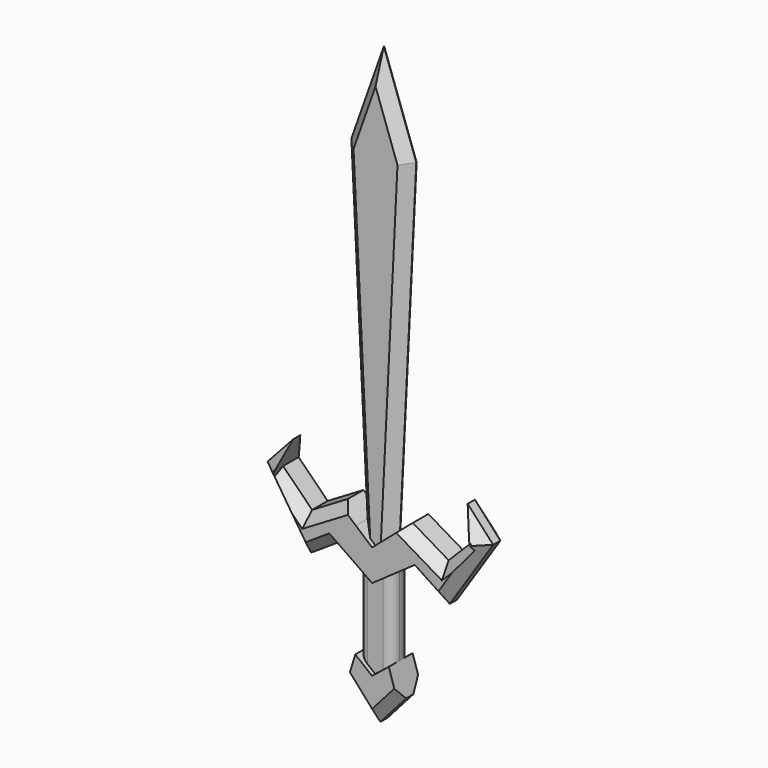
from build123d import *

# Parameters (mm, degrees)
F1_DEPTH      = 2.33167
F2_SIZE       = 2.286
F3_DEPTH      = 3.27792
F4_T4_DEPTH   = 23.2837004238
F4_T9_DEPTH   = 15.3016603011
F4_T14_DEPTH  = 15.3016603011
F4_T19_DEPTH  = 23.2837004238
F4_T24_DEPTH  = 23.2837004238
F4_T29_DEPTH  = 15.3016603011
F4_T34_DEPTH  = 23.2837004238
F4_T39_DEPTH  = 15.3016603011
F4_T44_DEPTH  = 20.0662153039
F4_T50_DEPTH  = 20.0662153039
F4_T56_DEPTH  = 20.0662153039
F4_T62_DEPTH  = 20.0662153039
F4_T68_DEPTH  = 20.8098338881
F4_T74_DEPTH  = 20.9196420642
F4_T80_DEPTH  = 20.9196420642
F4_T86_DEPTH  = 20.8098338881
F4_T93_DEPTH  = 20.0662153039
F4_T97_DEPTH  = 23.2837004238
F4_T104_DEPTH = 29.1625677342
F4_T108_DEPTH = 21.1805276116
F4_T115_DEPTH = 21.1805276116
F4_T119_DEPTH = 29.1625677342
F4_T126_DEPTH = 23.2837004238
F4_T130_DEPTH = 20.0662153039
F4_T137_DEPTH = 20.0662153039
F4_T141_DEPTH = 23.2837004238
F4_T148_DEPTH = 29.1625677342
F4_T152_DEPTH = 21.1805276116
F4_T159_DEPTH = 21.1805276116
F4_T163_DEPTH = 29.1625677342
F4_T170_DEPTH = 23.2837004238
F4_T174_DEPTH = 20.0662153039
F4_T181_DEPTH = 20.8098338881
F4_T185_DEPTH = 20.9196420642
F4_T192_DEPTH = 20.9196420642
F4_T196_DEPTH = 20.8098338881
F5_DEPTH      = 2.39562
F6_R          = 2.032
F7_DEPTH      = 3.2766
F8_SIZE       = 2.286


# Not quite as in the source:
# - a fillet or chamfer that OpenCascade refuses, or shapes differently, is made with other operations: its cross-section is extruded or revolved along the edge and cut away or added


with BuildPart() as f1:
    # F0 (on Front) → F1 (new body, symmetric)
    with BuildSketch(Plane.XZ):
        Polygon((0, -27.3264925927), (3.569676308, -24.2491848767), (7.1393526159, 48.2521876693), (0, 68.4393197298), (-7.1393526159, 48.2521876693), (-3.569676308, -24.2491848767), align=None)
    extrude(amount=F1_DEPTH, both=True)

    # F2
    f2_edges = [f1.edges().sort_by_distance(p)[0] for p in [
        (-5.354514, -2.33167, 12.001501),
        (5.354514, -2.33167, 12.001501),
        (-3.569676, -2.33167, 58.345754),
        (3.569676, -2.33167, 58.345754),
        (-3.569676, 2.33167, 58.345754),
        (3.569676, 2.33167, 58.345754),
        (5.354514, 2.33167, 12.001501),
        (-5.354514, 2.33167, 12.001501),
    ]]
    chamfer(f2_edges, length=F2_SIZE)

    # F0 (on Front) → F3 (join, symmetric)
    with BuildSketch(Plane.XZ):
        Polygon((-3.6927689798, -31.6347228363), (0, -34.2196598649), (3.6927689798, -31.6347228363), (7.3855379596, -29.0497858077), (15.2634456754, -34.2196598649), (24.812715756, -19.6683830609), (19.2023981363, -13.540154323), (21.41806297, -19.4485839456), (15.01726266, -25.849385187), (7.1393526159, -21.1718771607), (3.569676308, -24.2491848767), (0, -27.3264925927), (-3.569676308, -24.2491848767), (-7.1393526159, -21.1718771607), (-15.01726266, -25.849385187), (-21.41806297, -19.4485839456), (-19.2023981363, -13.540154323), (-24.812715756, -19.6683830609), (-15.2634456754, -34.2196598649), (-7.3855379596, -29.0497858077), align=None)
    extrude(amount=F3_DEPTH, both=True)

    # F4: chamfer of 2.286 on 16 edges, made by hand


with BuildPart() as f4_tool2:
    # F4_s3 → F4_t4 (new body)
    with BuildSketch(Plane(origin=(-1.6727458566, 0, 2.5489474878), x_dir=(0, 1, 0), z_dir=(0.5486562278, 0, -0.8360480511))):
        with BuildLine():
            Line((-3.3425778441, -29.1851456624), (-0.9272621559, -31.6004613506))
            Line((-0.9272621559, -31.6004613506), (-0.9272621559, -31.6461813506))
            ThreePointArc((-0.9272621559, -31.6461813506), (-2.102591078, -31.5815235065), (-3.27792, -31.5815235065))
            Line((-3.27792, -31.5815235065), (-3.32364, -31.5358035065))
            ThreePointArc((-3.32364, -31.5358035065), (-3.32364, -30.3604745845), (-3.3882978441, -29.1851456624))
            Line((-3.3882978441, -29.1851456624), (-3.3425778441, -29.1851456624))
        make_face()
    extrude(amount=F4_T4_DEPTH)

    split(bisect_by=Plane(origin=(-3.7030026198, 0, 3.3900531022), x_dir=(0, 1, 0), z_dir=(0.7375871681, 0, -0.6752519304)), keep=Keep.TOP)


with BuildPart() as f1_1:
    add(f1.part)

    # F4_t1: cut F4_tool2
    add(f4_tool2.part, mode=Mode.SUBTRACT)


with BuildPart() as f4_tool7:
    # F4_s8 → F4_t9 (new body)
    with BuildSketch(Plane(origin=(-26.3654470614, 0, -17.3023149911), x_dir=(0, 1, 0), z_dir=(0.8360480511, 0, 0.5486562278))):
        with BuildLine():
            Line((-3.3425778441, -17.8842375684), (-0.9272621559, -20.2995532566))
            Line((-0.9272621559, -20.2995532566), (-0.9272621559, -20.3452732566))
            ThreePointArc((-0.9272621559, -20.3452732566), (-2.102591078, -20.2806154125), (-3.27792, -20.2806154125))
            Line((-3.27792, -20.2806154125), (-3.32364, -20.2348954125))
            ThreePointArc((-3.32364, -20.2348954125), (-3.32364, -19.0595664905), (-3.3882978441, -17.8842375684))
            Line((-3.3882978441, -17.8842375684), (-3.3425778441, -17.8842375684))
        make_face()
    extrude(amount=F4_T9_DEPTH)

    split(bisect_by=Plane(origin=(-16.0763475957, 0, -22.9662220215), x_dir=(0, 1, 0), z_dir=(-0.5734621572, 0, -0.8192320516)), keep=Keep.TOP)


with BuildPart() as f1_2:
    add(f1_1.part)

    # F4_t6: cut F4_tool7
    add(f4_tool7.part, mode=Mode.SUBTRACT)


with BuildPart() as f4_tool12:
    # F4_s13 → F4_t14 (new body)
    with BuildSketch(Plane(origin=(13.5725237881, 0, -8.9069637719), x_dir=(0, 1, 0), z_dir=(0.8360480511, 0, -0.5486562278))):
        with BuildLine():
            Line((-3.3425778441, -17.8842375684), (-0.9272621559, -20.2995532566))
            Line((-0.9272621559, -20.2995532566), (-0.9272621559, -20.3452732566))
            ThreePointArc((-0.9272621559, -20.3452732566), (-2.102591078, -20.2806154125), (-3.27792, -20.2806154125))
            Line((-3.27792, -20.2806154125), (-3.32364, -20.2348954125))
            ThreePointArc((-3.32364, -20.2348954125), (-3.32364, -19.0595664905), (-3.3882978441, -17.8842375684))
            Line((-3.3882978441, -17.8842375684), (-3.3425778441, -17.8842375684))
        make_face()
    extrude(amount=F4_T14_DEPTH)

    split(bisect_by=Plane(origin=(16.0763475957, 0, -22.9662220215), x_dir=(0, 1, 0), z_dir=(0.5734621572, 0, -0.8192320516)), keep=Keep.TOP)


with BuildPart() as f1_3:
    add(f1_2.part)

    # F4_t11: cut F4_tool12
    add(f4_tool12.part, mode=Mode.SUBTRACT)


with BuildPart() as f4_tool17:
    # F4_s18 → F4_t19 (new body)
    with BuildSketch(Plane(origin=(-11.102001386, 0, -16.9173448738), x_dir=(0, 1, 0), z_dir=(0.5486562278, 0, 0.8360480511))):
        with BuildLine():
            Line((-3.3425778441, -29.1851456624), (-0.9272621559, -31.6004613506))
            Line((-0.9272621559, -31.6004613506), (-0.9272621559, -31.6461813506))
            ThreePointArc((-0.9272621559, -31.6461813506), (-2.102591078, -31.5815235065), (-3.27792, -31.5815235065))
            Line((-3.27792, -31.5815235065), (-3.32364, -31.5358035065))
            ThreePointArc((-3.32364, -31.5358035065), (-3.32364, -30.3604745845), (-3.3882978441, -29.1851456624))
            Line((-3.3882978441, -29.1851456624), (-3.3425778441, -29.1851456624))
        make_face()
    extrude(amount=F4_T19_DEPTH)

    split(bisect_by=Plane(origin=(3.7030026198, 0, 3.3900531022), x_dir=(0, 1, 0), z_dir=(-0.7375871681, 0, -0.6752519304)), keep=Keep.TOP)


with BuildPart() as f1_4:
    add(f1_3.part)

    # F4_t16: cut F4_tool17
    add(f4_tool17.part, mode=Mode.SUBTRACT)


with BuildPart() as f4_tool22:
    # F4_s23 → F4_t24 (new body)
    with BuildSketch(Plane(origin=(-1.6727458566, 0, 2.5489474878), x_dir=(0, 1, 0), z_dir=(0.5486562278, 0, -0.8360480511))):
        with BuildLine():
            Line((3.3425778441, -29.1851456624), (0.9272621559, -31.6004613506))
            Line((0.9272621559, -31.6004613506), (0.9272621559, -31.6461813506))
            ThreePointArc((0.9272621559, -31.6461813506), (2.102591078, -31.5815235065), (3.27792, -31.5815235065))
            Line((3.27792, -31.5815235065), (3.32364, -31.5358035065))
            ThreePointArc((3.32364, -31.5358035065), (3.32364, -30.3604745845), (3.3882978441, -29.1851456624))
            Line((3.3882978441, -29.1851456624), (3.3425778441, -29.1851456624))
        make_face()
    extrude(amount=F4_T24_DEPTH)

    split(bisect_by=Plane(origin=(-3.7030026198, 0, 3.3900531022), x_dir=(0, 1, 0), z_dir=(0.7375871681, 0, -0.6752519304)), keep=Keep.TOP)


with BuildPart() as f1_5:
    add(f1_4.part)

    # F4_t21: cut F4_tool22
    add(f4_tool22.part, mode=Mode.SUBTRACT)


with BuildPart() as f4_tool27:
    # F4_s28 → F4_t29 (new body)
    with BuildSketch(Plane(origin=(-26.3654470614, 0, -17.3023149911), x_dir=(0, 1, 0), z_dir=(0.8360480511, 0, 0.5486562278))):
        with BuildLine():
            Line((3.3425778441, -17.8842375684), (0.9272621559, -20.2995532566))
            Line((0.9272621559, -20.2995532566), (0.9272621559, -20.3452732566))
            ThreePointArc((0.9272621559, -20.3452732566), (2.102591078, -20.2806154125), (3.27792, -20.2806154125))
            Line((3.27792, -20.2806154125), (3.32364, -20.2348954125))
            ThreePointArc((3.32364, -20.2348954125), (3.32364, -19.0595664905), (3.3882978441, -17.8842375684))
            Line((3.3882978441, -17.8842375684), (3.3425778441, -17.8842375684))
        make_face()
    extrude(amount=F4_T29_DEPTH)

    split(bisect_by=Plane(origin=(-16.0763475957, 0, -22.9662220215), x_dir=(0, 1, 0), z_dir=(-0.5734621572, 0, -0.8192320516)), keep=Keep.TOP)


with BuildPart() as f1_6:
    add(f1_5.part)

    # F4_t26: cut F4_tool27
    add(f4_tool27.part, mode=Mode.SUBTRACT)


with BuildPart() as f4_tool32:
    # F4_s33 → F4_t34 (new body)
    with BuildSketch(Plane(origin=(-11.102001386, 0, -16.9173448738), x_dir=(0, 1, 0), z_dir=(0.5486562278, 0, 0.8360480511))):
        with BuildLine():
            Line((3.3425778441, -29.1851456624), (0.9272621559, -31.6004613506))
            Line((0.9272621559, -31.6004613506), (0.9272621559, -31.6461813506))
            ThreePointArc((0.9272621559, -31.6461813506), (2.102591078, -31.5815235065), (3.27792, -31.5815235065))
            Line((3.27792, -31.5815235065), (3.32364, -31.5358035065))
            ThreePointArc((3.32364, -31.5358035065), (3.32364, -30.3604745845), (3.3882978441, -29.1851456624))
            Line((3.3882978441, -29.1851456624), (3.3425778441, -29.1851456624))
        make_face()
    extrude(amount=F4_T34_DEPTH)

    split(bisect_by=Plane(origin=(3.7030026198, 0, 3.3900531022), x_dir=(0, 1, 0), z_dir=(-0.7375871681, 0, -0.6752519304)), keep=Keep.TOP)


with BuildPart() as f1_7:
    add(f1_6.part)

    # F4_t31: cut F4_tool32
    add(f4_tool32.part, mode=Mode.SUBTRACT)


with BuildPart() as f4_tool37:
    # F4_s38 → F4_t39 (new body)
    with BuildSketch(Plane(origin=(13.5725237881, 0, -8.9069637719), x_dir=(0, 1, 0), z_dir=(0.8360480511, 0, -0.5486562278))):
        with BuildLine():
            Line((3.3425778441, -17.8842375684), (0.9272621559, -20.2995532566))
            Line((0.9272621559, -20.2995532566), (0.9272621559, -20.3452732566))
            ThreePointArc((0.9272621559, -20.3452732566), (2.102591078, -20.2806154125), (3.27792, -20.2806154125))
            Line((3.27792, -20.2806154125), (3.32364, -20.2348954125))
            ThreePointArc((3.32364, -20.2348954125), (3.32364, -19.0595664905), (3.3882978441, -17.8842375684))
            Line((3.3882978441, -17.8842375684), (3.3425778441, -17.8842375684))
        make_face()
    extrude(amount=F4_T39_DEPTH)

    split(bisect_by=Plane(origin=(16.0763475957, 0, -22.9662220215), x_dir=(0, 1, 0), z_dir=(0.5734621572, 0, -0.8192320516)), keep=Keep.TOP)


with BuildPart() as f1_8:
    add(f1_7.part)

    # F4_t36: cut F4_tool37
    add(f4_tool37.part, mode=Mode.SUBTRACT)


with BuildPart() as f4_tool42:
    # F4_s43 → F4_t44 (new body)
    with BuildSketch(Plane(origin=(-11.5296790165, 0, -12.5940303342), x_dir=(0, 1, 0), z_dir=(-0.6752519304, 0, -0.7375871681))):
        with BuildLine():
            Line((3.3425778441, -2.6697692731), (0.9272621559, -5.0850849612))
            Line((0.9272621559, -5.0850849612), (0.9272621559, -5.1308049612))
            ThreePointArc((0.9272621559, -5.1308049612), (2.102591078, -5.0661471171), (3.27792, -5.0661471171))
            Line((3.27792, -5.0661471171), (3.32364, -5.0204271171))
            ThreePointArc((3.32364, -5.0204271171), (3.32364, -3.8450981951), (3.3882978441, -2.6697692731))
            Line((3.3882978441, -2.6697692731), (3.3425778441, -2.6697692731))
        make_face()
    extrude(amount=F4_T44_DEPTH)

    split(bisect_by=Plane(origin=(-12.3834089838, 0, 4.6437861767), x_dir=(0, 1, 0), z_dir=(-0.9363289835, 0, 0.3511239592)), keep=Keep.TOP)

    split(bisect_by=Plane(origin=(-26.3654470614, 0, -17.3023149911), x_dir=(0, 1, 0), z_dir=(0.8360480511, 0, 0.5486562278)), keep=Keep.TOP)


with BuildPart() as f1_9:
    add(f1_8.part)

    # F4_t41: cut F4_tool42
    add(f4_tool42.part, mode=Mode.SUBTRACT)


with BuildPart() as f4_tool48:
    # F4_s49 → F4_t50 (new body)
    with BuildSketch(Plane(origin=(-11.5296790165, 0, -12.5940303342), x_dir=(0, 1, 0), z_dir=(-0.6752519304, 0, -0.7375871681))):
        with BuildLine():
            Line((-3.3425778441, -2.6697692731), (-0.9272621559, -5.0850849612))
            Line((-0.9272621559, -5.0850849612), (-0.9272621559, -5.1308049612))
            ThreePointArc((-0.9272621559, -5.1308049612), (-2.102591078, -5.0661471171), (-3.27792, -5.0661471171))
            Line((-3.27792, -5.0661471171), (-3.32364, -5.0204271171))
            ThreePointArc((-3.32364, -5.0204271171), (-3.32364, -3.8450981951), (-3.3882978441, -2.6697692731))
            Line((-3.3882978441, -2.6697692731), (-3.3425778441, -2.6697692731))
        make_face()
    extrude(amount=F4_T50_DEPTH)

    split(bisect_by=Plane(origin=(-12.3834089838, 0, 4.6437861767), x_dir=(0, 1, 0), z_dir=(-0.9363289835, 0, 0.3511239592)), keep=Keep.TOP)

    split(bisect_by=Plane(origin=(-26.3654470614, 0, -17.3023149911), x_dir=(0, 1, 0), z_dir=(0.8360480511, 0, 0.5486562278)), keep=Keep.TOP)


with BuildPart() as f1_10:
    add(f1_9.part)

    # F4_t47: cut F4_tool48
    add(f4_tool48.part, mode=Mode.SUBTRACT)


with BuildPart() as f4_tool54:
    # F4_s55 → F4_t56 (new body)
    with BuildSketch(Plane(origin=(25.0794296361, 0, -27.3946132541), x_dir=(0, 1, 0), z_dir=(-0.6752519304, 0, 0.7375871681))):
        with BuildLine():
            Line((3.3425778441, -2.6697692731), (0.9272621559, -5.0850849612))
            Line((0.9272621559, -5.0850849612), (0.9272621559, -5.1308049612))
            ThreePointArc((0.9272621559, -5.1308049612), (2.102591078, -5.0661471171), (3.27792, -5.0661471171))
            Line((3.27792, -5.0661471171), (3.32364, -5.0204271171))
            ThreePointArc((3.32364, -5.0204271171), (3.32364, -3.8450981951), (3.3882978441, -2.6697692731))
            Line((3.3882978441, -2.6697692731), (3.3425778441, -2.6697692731))
        make_face()
    extrude(amount=F4_T56_DEPTH)

    split(bisect_by=Plane(origin=(12.3834089838, 0, 4.6437861767), x_dir=(0, 1, 0), z_dir=(0.9363289835, 0, 0.3511239592)), keep=Keep.TOP)

    split(bisect_by=Plane(origin=(26.3654470614, 0, -17.3023149911), x_dir=(0, 1, 0), z_dir=(-0.8360480511, 0, 0.5486562278)), keep=Keep.TOP)


with BuildPart() as f1_11:
    add(f1_10.part)

    # F4_t53: cut F4_tool54
    add(f4_tool54.part, mode=Mode.SUBTRACT)


with BuildPart() as f4_tool60:
    # F4_s61 → F4_t62 (new body)
    with BuildSketch(Plane(origin=(25.0794296361, 0, -27.3946132541), x_dir=(0, 1, 0), z_dir=(-0.6752519304, 0, 0.7375871681))):
        with BuildLine():
            Line((-3.3425778441, -2.6697692731), (-0.9272621559, -5.0850849612))
            Line((-0.9272621559, -5.0850849612), (-0.9272621559, -5.1308049612))
            ThreePointArc((-0.9272621559, -5.1308049612), (-2.102591078, -5.0661471171), (-3.27792, -5.0661471171))
            Line((-3.27792, -5.0661471171), (-3.32364, -5.0204271171))
            ThreePointArc((-3.32364, -5.0204271171), (-3.32364, -3.8450981951), (-3.3882978441, -2.6697692731))
            Line((-3.3882978441, -2.6697692731), (-3.3425778441, -2.6697692731))
        make_face()
    extrude(amount=F4_T62_DEPTH)

    split(bisect_by=Plane(origin=(12.3834089838, 0, 4.6437861767), x_dir=(0, 1, 0), z_dir=(0.9363289835, 0, 0.3511239592)), keep=Keep.TOP)

    split(bisect_by=Plane(origin=(26.3654470614, 0, -17.3023149911), x_dir=(0, 1, 0), z_dir=(-0.8360480511, 0, 0.5486562278)), keep=Keep.TOP)


with BuildPart() as f1_12:
    add(f1_11.part)

    # F4_t59: cut F4_tool60
    add(f4_tool60.part, mode=Mode.SUBTRACT)


with BuildPart() as f4_tool66:
    # F4_s67 → F4_t68 (new body)
    with BuildSketch(Plane(origin=(5.1417245926, 0, 5.1417253407), x_dir=(0, 1, 0), z_dir=(-0.7071067297, 0, -0.7071068326))):
        with BuildLine():
            Line((-3.3425778441, 31.2477411038), (-0.9272621559, 28.8324254157))
            Line((-0.9272621559, 28.8324254157), (-0.9272621559, 28.7867054157))
            ThreePointArc((-0.9272621559, 28.7867054157), (-2.102591078, 28.8513632597), (-3.27792, 28.8513632597))
            Line((-3.27792, 28.8513632597), (-3.32364, 28.8970832597))
            ThreePointArc((-3.32364, 28.8970832597), (-3.32364, 30.0724121818), (-3.3882978441, 31.2477411038))
            Line((-3.3882978441, 31.2477411038), (-3.3425778441, 31.2477411038))
        make_face()
    extrude(amount=F4_T68_DEPTH)

    split(bisect_by=Plane(origin=(12.3834089838, 0, 4.6437861767), x_dir=(0, 1, 0), z_dir=(-0.9363289835, 0, -0.3511239592)), keep=Keep.TOP)

    split(bisect_by=Plane(origin=(-7.4333534191, 0, -12.5193349174), x_dir=(0, 1, 0), z_dir=(0.5105386684, 0, 0.8598547947)), keep=Keep.TOP)


with BuildPart() as f1_13:
    add(f1_12.part)

    # F4_t65: cut F4_tool66
    add(f4_tool66.part, mode=Mode.SUBTRACT)


with BuildPart() as f4_tool72:
    # F4_s73 → F4_t74 (new body)
    with BuildSketch(Plane(origin=(27.5055883236, 0, -16.3314393582), x_dir=(0, 1, 0), z_dir=(-0.8598547947, 0, 0.5105386684))):
        with BuildLine():
            Line((-3.3425778441, 16.9104823563), (-0.9272621559, 14.4951666682))
            Line((-0.9272621559, 14.4951666682), (-0.9272621559, 14.4494466682))
            ThreePointArc((-0.9272621559, 14.4494466682), (-2.102591078, 14.5141045123), (-3.27792, 14.5141045123))
            Line((-3.27792, 14.5141045123), (-3.32364, 14.5598245123))
            ThreePointArc((-3.32364, 14.5598245123), (-3.32364, 15.7351534343), (-3.3882978441, 16.9104823563))
            Line((-3.3882978441, 16.9104823563), (-3.3425778441, 16.9104823563))
        make_face()
    extrude(amount=F4_T74_DEPTH)

    split(bisect_by=Plane(origin=(13.5141252764, 0, -15.6763824986), x_dir=(0, 1, 0), z_dir=(0.6529396895, 0, -0.7574099035)), keep=Keep.TOP)

    split(bisect_by=Plane(origin=(20.433325016, 0, -20.4333220429), x_dir=(0, 1, 0), z_dir=(-0.7071068326, 0, 0.7071067297)), keep=Keep.TOP)


with BuildPart() as f1_14:
    add(f1_13.part)

    # F4_t71: cut F4_tool72
    add(f4_tool72.part, mode=Mode.SUBTRACT)


with BuildPart() as f4_tool78:
    # F4_s79 → F4_t80 (new body)
    with BuildSketch(Plane(origin=(-9.5177337904, 0, -5.6511531547), x_dir=(0, 1, 0), z_dir=(-0.8598547947, 0, -0.5105386684))):
        with BuildLine():
            Line((-3.3425778441, 16.9104823563), (-0.9272621559, 14.4951666682))
            Line((-0.9272621559, 14.4951666682), (-0.9272621559, 14.4494466682))
            ThreePointArc((-0.9272621559, 14.4494466682), (-2.102591078, 14.5141045123), (-3.27792, 14.5141045123))
            Line((-3.27792, 14.5141045123), (-3.32364, 14.5598245123))
            ThreePointArc((-3.32364, 14.5598245123), (-3.32364, 15.7351534343), (-3.3882978441, 16.9104823563))
            Line((-3.3882978441, 16.9104823563), (-3.3425778441, 16.9104823563))
        make_face()
    extrude(amount=F4_T80_DEPTH)

    split(bisect_by=Plane(origin=(-13.5141252764, 0, -15.6763824986), x_dir=(0, 1, 0), z_dir=(-0.6529396895, 0, -0.7574099035)), keep=Keep.TOP)

    split(bisect_by=Plane(origin=(-20.433325016, 0, -20.4333220429), x_dir=(0, 1, 0), z_dir=(0.7071068326, 0, 0.7071067297)), keep=Keep.TOP)


with BuildPart() as f1_15:
    add(f1_14.part)

    # F4_t77: cut F4_tool78
    add(f4_tool78.part, mode=Mode.SUBTRACT)


with BuildPart() as f4_tool84:
    # F4_s85 → F4_t86 (new body)
    with BuildSketch(Plane(origin=(9.5730489946, 0, -9.5730503875), x_dir=(0, 1, 0), z_dir=(-0.7071067297, 0, 0.7071068326))):
        with BuildLine():
            Line((-3.3425778441, 31.2477411038), (-0.9272621559, 28.8324254157))
            Line((-0.9272621559, 28.8324254157), (-0.9272621559, 28.7867054157))
            ThreePointArc((-0.9272621559, 28.7867054157), (-2.102591078, 28.8513632597), (-3.27792, 28.8513632597))
            Line((-3.27792, 28.8513632597), (-3.32364, 28.8970832597))
            ThreePointArc((-3.32364, 28.8970832597), (-3.32364, 30.0724121818), (-3.3882978441, 31.2477411038))
            Line((-3.3882978441, 31.2477411038), (-3.3425778441, 31.2477411038))
        make_face()
    extrude(amount=F4_T86_DEPTH)

    split(bisect_by=Plane(origin=(-12.3834089838, 0, 4.6437861767), x_dir=(0, 1, 0), z_dir=(0.9363289835, 0, -0.3511239592)), keep=Keep.TOP)

    split(bisect_by=Plane(origin=(7.4333534191, 0, -12.5193349174), x_dir=(0, 1, 0), z_dir=(-0.5105386684, 0, 0.8598547947)), keep=Keep.TOP)


with BuildPart() as f1_16:
    add(f1_15.part)

    # F4_t83: cut F4_tool84
    add(f4_tool84.part, mode=Mode.SUBTRACT)


with BuildPart() as f4_tool91:
    # F4_s92 → F4_t93 (new body)
    with BuildSketch(Plane(origin=(-11.5296790165, 0, -12.5940303342), x_dir=(0, 1, 0), z_dir=(-0.6752519304, 0, -0.7375871681))):
        with BuildLine():
            Line((-3.3425778441, -2.6697692731), (-0.9272621559, -5.0850849612))
            Line((-0.9272621559, -5.0850849612), (-0.9272621559, -5.1308049612))
            ThreePointArc((-0.9272621559, -5.1308049612), (-2.102591078, -5.0661471171), (-3.27792, -5.0661471171))
            Line((-3.27792, -5.0661471171), (-3.32364, -5.0204271171))
            ThreePointArc((-3.32364, -5.0204271171), (-3.32364, -3.8450981951), (-3.3882978441, -2.6697692731))
            Line((-3.3882978441, -2.6697692731), (-3.3425778441, -2.6697692731))
        make_face()
    extrude(amount=F4_T93_DEPTH)

    split(bisect_by=Plane(origin=(-26.3654470614, 0, -17.3023149911), x_dir=(0, 1, 0), z_dir=(-0.8360480511, 0, -0.5486562278)), keep=Keep.TOP)


with BuildPart() as f4_tool95:
    # F4_s96 → F4_t97 (new body)
    with BuildSketch(Plane(origin=(-1.6727458566, 0, 2.5489474878), x_dir=(0, 1, 0), z_dir=(0.5486562278, 0, -0.8360480511))):
        with BuildLine():
            Line((-3.3425778441, -29.1851456624), (-0.9272621559, -31.6004613506))
            Line((-0.9272621559, -31.6004613506), (-0.9272621559, -31.6461813506))
            ThreePointArc((-0.9272621559, -31.6461813506), (-2.102591078, -31.5815235065), (-3.27792, -31.5815235065))
            Line((-3.27792, -31.5815235065), (-3.32364, -31.5358035065))
            ThreePointArc((-3.32364, -31.5358035065), (-3.32364, -30.3604745845), (-3.3882978441, -29.1851456624))
            Line((-3.3882978441, -29.1851456624), (-3.3425778441, -29.1851456624))
        make_face()
    extrude(amount=F4_T97_DEPTH)

    split(bisect_by=Plane(origin=(-3.7030026198, 0, 3.3900531022), x_dir=(0, 1, 0), z_dir=(-0.7375871681, 0, 0.6752519304)), keep=Keep.TOP)


with BuildPart() as f4_tool91_1:
    add(f4_tool91.part)

    # F4_t99: intersect F4_tool95
    add(f4_tool95.part, mode=Mode.INTERSECT)


with BuildPart() as f1_17:
    add(f1_16.part)

    # F4_t89: cut F4_tool91
    add(f4_tool91_1.part, mode=Mode.SUBTRACT)


with BuildPart() as f4_tool102:
    # F4_s103 → F4_t104 (new body)
    with BuildSketch(Plane(origin=(-1.6727458566, 0, 2.5489474878), x_dir=(0, 1, 0), z_dir=(0.5486562278, 0, -0.8360480511))):
        with BuildLine():
            Line((-3.3425778441, -29.1851456624), (-0.9272621559, -31.6004613506))
            Line((-0.9272621559, -31.6004613506), (-0.9272621559, -31.6461813506))
            ThreePointArc((-0.9272621559, -31.6461813506), (-2.102591078, -31.5815235065), (-3.27792, -31.5815235065))
            Line((-3.27792, -31.5815235065), (-3.32364, -31.5358035065))
            ThreePointArc((-3.32364, -31.5358035065), (-3.32364, -30.3604745845), (-3.3882978441, -29.1851456624))
            Line((-3.3882978441, -29.1851456624), (-3.3425778441, -29.1851456624))
        make_face()
    extrude(amount=F4_T104_DEPTH)

    split(bisect_by=Plane(origin=(11.102001386, 0, -16.9173448738), x_dir=(0, 1, 0), z_dir=(0.5486562278, 0, -0.8360480511)), keep=Keep.TOP)


with BuildPart() as f4_tool106:
    # F4_s107 → F4_t108 (new body)
    with BuildSketch(Plane(origin=(-31.280462619, 0, -20.5277921532), x_dir=(0, 1, 0), z_dir=(0.8360480511, 0, 0.5486562278))):
        with BuildLine():
            Line((-3.3425778441, -17.8842375684), (-0.9272621559, -20.2995532566))
            Line((-0.9272621559, -20.2995532566), (-0.9272621559, -20.3452732566))
            ThreePointArc((-0.9272621559, -20.3452732566), (-2.102591078, -20.2806154125), (-3.27792, -20.2806154125))
            Line((-3.27792, -20.2806154125), (-3.32364, -20.2348954125))
            ThreePointArc((-3.32364, -20.2348954125), (-3.32364, -19.0595664905), (-3.3882978441, -17.8842375684))
            Line((-3.3882978441, -17.8842375684), (-3.3425778441, -17.8842375684))
        make_face()
    extrude(amount=F4_T108_DEPTH)

    split(bisect_by=Plane(origin=(-26.3654470614, 0, -17.3023149911), x_dir=(0, 1, 0), z_dir=(-0.8360480511, 0, -0.5486562278)), keep=Keep.TOP)


with BuildPart() as f4_tool102_1:
    add(f4_tool102.part)

    # F4_t110: intersect F4_tool106
    add(f4_tool106.part, mode=Mode.INTERSECT)


with BuildPart() as f1_18:
    add(f1_17.part)

    # F4_t100: cut F4_tool102
    add(f4_tool102_1.part, mode=Mode.SUBTRACT)


with BuildPart() as f4_tool113:
    # F4_s114 → F4_t115 (new body)
    with BuildSketch(Plane(origin=(13.5725237881, 0, -8.9069637719), x_dir=(0, 1, 0), z_dir=(0.8360480511, 0, -0.5486562278))):
        with BuildLine():
            Line((-3.3425778441, -17.8842375684), (-0.9272621559, -20.2995532566))
            Line((-0.9272621559, -20.2995532566), (-0.9272621559, -20.3452732566))
            ThreePointArc((-0.9272621559, -20.3452732566), (-2.102591078, -20.2806154125), (-3.27792, -20.2806154125))
            Line((-3.27792, -20.2806154125), (-3.32364, -20.2348954125))
            ThreePointArc((-3.32364, -20.2348954125), (-3.32364, -19.0595664905), (-3.3882978441, -17.8842375684))
            Line((-3.3882978441, -17.8842375684), (-3.3425778441, -17.8842375684))
        make_face()
    extrude(amount=F4_T115_DEPTH)

    split(bisect_by=Plane(origin=(26.3654470614, 0, -17.3023149911), x_dir=(0, 1, 0), z_dir=(0.8360480511, 0, -0.5486562278)), keep=Keep.TOP)


with BuildPart() as f4_tool117:
    # F4_s118 → F4_t119 (new body)
    with BuildSketch(Plane(origin=(-14.3274785481, 0, -21.8323604314), x_dir=(0, 1, 0), z_dir=(0.5486562278, 0, 0.8360480511))):
        with BuildLine():
            Line((-3.3425778441, -29.1851456624), (-0.9272621559, -31.6004613506))
            Line((-0.9272621559, -31.6004613506), (-0.9272621559, -31.6461813506))
            ThreePointArc((-0.9272621559, -31.6461813506), (-2.102591078, -31.5815235065), (-3.27792, -31.5815235065))
            Line((-3.27792, -31.5815235065), (-3.32364, -31.5358035065))
            ThreePointArc((-3.32364, -31.5358035065), (-3.32364, -30.3604745845), (-3.3882978441, -29.1851456624))
            Line((-3.3882978441, -29.1851456624), (-3.3425778441, -29.1851456624))
        make_face()
    extrude(amount=F4_T119_DEPTH)

    split(bisect_by=Plane(origin=(-11.102001386, 0, -16.9173448738), x_dir=(0, 1, 0), z_dir=(-0.5486562278, 0, -0.8360480511)), keep=Keep.TOP)


with BuildPart() as f4_tool113_1:
    add(f4_tool113.part)

    # F4_t121: intersect F4_tool117
    add(f4_tool117.part, mode=Mode.INTERSECT)


with BuildPart() as f1_19:
    add(f1_18.part)

    # F4_t111: cut F4_tool113
    add(f4_tool113_1.part, mode=Mode.SUBTRACT)


with BuildPart() as f4_tool124:
    # F4_s125 → F4_t126 (new body)
    with BuildSketch(Plane(origin=(-11.102001386, 0, -16.9173448738), x_dir=(0, 1, 0), z_dir=(0.5486562278, 0, 0.8360480511))):
        with BuildLine():
            Line((-3.3425778441, -29.1851456624), (-0.9272621559, -31.6004613506))
            Line((-0.9272621559, -31.6004613506), (-0.9272621559, -31.6461813506))
            ThreePointArc((-0.9272621559, -31.6461813506), (-2.102591078, -31.5815235065), (-3.27792, -31.5815235065))
            Line((-3.27792, -31.5815235065), (-3.32364, -31.5358035065))
            ThreePointArc((-3.32364, -31.5358035065), (-3.32364, -30.3604745845), (-3.3882978441, -29.1851456624))
            Line((-3.3882978441, -29.1851456624), (-3.3425778441, -29.1851456624))
        make_face()
    extrude(amount=F4_T126_DEPTH)

    split(bisect_by=Plane(origin=(3.7030026198, 0, 3.3900531022), x_dir=(0, 1, 0), z_dir=(0.7375871681, 0, 0.6752519304)), keep=Keep.TOP)


with BuildPart() as f4_tool128:
    # F4_s129 → F4_t130 (new body)
    with BuildSketch(Plane(origin=(25.0794296361, 0, -27.3946132541), x_dir=(0, 1, 0), z_dir=(-0.6752519304, 0, 0.7375871681))):
        with BuildLine():
            Line((-3.3425778441, -2.6697692731), (-0.9272621559, -5.0850849612))
            Line((-0.9272621559, -5.0850849612), (-0.9272621559, -5.1308049612))
            ThreePointArc((-0.9272621559, -5.1308049612), (-2.102591078, -5.0661471171), (-3.27792, -5.0661471171))
            Line((-3.27792, -5.0661471171), (-3.32364, -5.0204271171))
            ThreePointArc((-3.32364, -5.0204271171), (-3.32364, -3.8450981951), (-3.3882978441, -2.6697692731))
            Line((-3.3882978441, -2.6697692731), (-3.3425778441, -2.6697692731))
        make_face()
    extrude(amount=F4_T130_DEPTH)

    split(bisect_by=Plane(origin=(26.3654470614, 0, -17.3023149911), x_dir=(0, 1, 0), z_dir=(0.8360480511, 0, -0.5486562278)), keep=Keep.TOP)


with BuildPart() as f4_tool124_1:
    add(f4_tool124.part)

    # F4_t132: intersect F4_tool128
    add(f4_tool128.part, mode=Mode.INTERSECT)


with BuildPart() as f1_20:
    add(f1_19.part)

    # F4_t122: cut F4_tool124
    add(f4_tool124_1.part, mode=Mode.SUBTRACT)


with BuildPart() as f4_tool135:
    # F4_s136 → F4_t137 (new body)
    with BuildSketch(Plane(origin=(-11.5296790165, 0, -12.5940303342), x_dir=(0, 1, 0), z_dir=(-0.6752519304, 0, -0.7375871681))):
        with BuildLine():
            Line((3.3425778441, -2.6697692731), (0.9272621559, -5.0850849612))
            Line((0.9272621559, -5.0850849612), (0.9272621559, -5.1308049612))
            ThreePointArc((0.9272621559, -5.1308049612), (2.102591078, -5.0661471171), (3.27792, -5.0661471171))
            Line((3.27792, -5.0661471171), (3.32364, -5.0204271171))
            ThreePointArc((3.32364, -5.0204271171), (3.32364, -3.8450981951), (3.3882978441, -2.6697692731))
            Line((3.3882978441, -2.6697692731), (3.3425778441, -2.6697692731))
        make_face()
    extrude(amount=F4_T137_DEPTH)

    split(bisect_by=Plane(origin=(-26.3654470614, 0, -17.3023149911), x_dir=(0, 1, 0), z_dir=(-0.8360480511, 0, -0.5486562278)), keep=Keep.TOP)


with BuildPart() as f4_tool139:
    # F4_s140 → F4_t141 (new body)
    with BuildSketch(Plane(origin=(-1.6727458566, 0, 2.5489474878), x_dir=(0, 1, 0), z_dir=(0.5486562278, 0, -0.8360480511))):
        with BuildLine():
            Line((3.3425778441, -29.1851456624), (0.9272621559, -31.6004613506))
            Line((0.9272621559, -31.6004613506), (0.9272621559, -31.6461813506))
            ThreePointArc((0.9272621559, -31.6461813506), (2.102591078, -31.5815235065), (3.27792, -31.5815235065))
            Line((3.27792, -31.5815235065), (3.32364, -31.5358035065))
            ThreePointArc((3.32364, -31.5358035065), (3.32364, -30.3604745845), (3.3882978441, -29.1851456624))
            Line((3.3882978441, -29.1851456624), (3.3425778441, -29.1851456624))
        make_face()
    extrude(amount=F4_T141_DEPTH)

    split(bisect_by=Plane(origin=(-3.7030026198, 0, 3.3900531022), x_dir=(0, 1, 0), z_dir=(-0.7375871681, 0, 0.6752519304)), keep=Keep.TOP)


with BuildPart() as f4_tool135_1:
    add(f4_tool135.part)

    # F4_t143: intersect F4_tool139
    add(f4_tool139.part, mode=Mode.INTERSECT)


with BuildPart() as f1_21:
    add(f1_20.part)

    # F4_t133: cut F4_tool135
    add(f4_tool135_1.part, mode=Mode.SUBTRACT)


with BuildPart() as f4_tool146:
    # F4_s147 → F4_t148 (new body)
    with BuildSketch(Plane(origin=(-1.6727458566, 0, 2.5489474878), x_dir=(0, 1, 0), z_dir=(0.5486562278, 0, -0.8360480511))):
        with BuildLine():
            Line((3.3425778441, -29.1851456624), (0.9272621559, -31.6004613506))
            Line((0.9272621559, -31.6004613506), (0.9272621559, -31.6461813506))
            ThreePointArc((0.9272621559, -31.6461813506), (2.102591078, -31.5815235065), (3.27792, -31.5815235065))
            Line((3.27792, -31.5815235065), (3.32364, -31.5358035065))
            ThreePointArc((3.32364, -31.5358035065), (3.32364, -30.3604745845), (3.3882978441, -29.1851456624))
            Line((3.3882978441, -29.1851456624), (3.3425778441, -29.1851456624))
        make_face()
    extrude(amount=F4_T148_DEPTH)

    split(bisect_by=Plane(origin=(11.102001386, 0, -16.9173448738), x_dir=(0, 1, 0), z_dir=(0.5486562278, 0, -0.8360480511)), keep=Keep.TOP)


with BuildPart() as f4_tool150:
    # F4_s151 → F4_t152 (new body)
    with BuildSketch(Plane(origin=(-31.280462619, 0, -20.5277921532), x_dir=(0, 1, 0), z_dir=(0.8360480511, 0, 0.5486562278))):
        with BuildLine():
            Line((3.3425778441, -17.8842375684), (0.9272621559, -20.2995532566))
            Line((0.9272621559, -20.2995532566), (0.9272621559, -20.3452732566))
            ThreePointArc((0.9272621559, -20.3452732566), (2.102591078, -20.2806154125), (3.27792, -20.2806154125))
            Line((3.27792, -20.2806154125), (3.32364, -20.2348954125))
            ThreePointArc((3.32364, -20.2348954125), (3.32364, -19.0595664905), (3.3882978441, -17.8842375684))
            Line((3.3882978441, -17.8842375684), (3.3425778441, -17.8842375684))
        make_face()
    extrude(amount=F4_T152_DEPTH)

    split(bisect_by=Plane(origin=(-26.3654470614, 0, -17.3023149911), x_dir=(0, 1, 0), z_dir=(-0.8360480511, 0, -0.5486562278)), keep=Keep.TOP)


with BuildPart() as f4_tool146_1:
    add(f4_tool146.part)

    # F4_t154: intersect F4_tool150
    add(f4_tool150.part, mode=Mode.INTERSECT)


with BuildPart() as f1_22:
    add(f1_21.part)

    # F4_t144: cut F4_tool146
    add(f4_tool146_1.part, mode=Mode.SUBTRACT)


with BuildPart() as f4_tool157:
    # F4_s158 → F4_t159 (new body)
    with BuildSketch(Plane(origin=(13.5725237881, 0, -8.9069637719), x_dir=(0, 1, 0), z_dir=(0.8360480511, 0, -0.5486562278))):
        with BuildLine():
            Line((3.3425778441, -17.8842375684), (0.9272621559, -20.2995532566))
            Line((0.9272621559, -20.2995532566), (0.9272621559, -20.3452732566))
            ThreePointArc((0.9272621559, -20.3452732566), (2.102591078, -20.2806154125), (3.27792, -20.2806154125))
            Line((3.27792, -20.2806154125), (3.32364, -20.2348954125))
            ThreePointArc((3.32364, -20.2348954125), (3.32364, -19.0595664905), (3.3882978441, -17.8842375684))
            Line((3.3882978441, -17.8842375684), (3.3425778441, -17.8842375684))
        make_face()
    extrude(amount=F4_T159_DEPTH)

    split(bisect_by=Plane(origin=(26.3654470614, 0, -17.3023149911), x_dir=(0, 1, 0), z_dir=(0.8360480511, 0, -0.5486562278)), keep=Keep.TOP)


with BuildPart() as f4_tool161:
    # F4_s162 → F4_t163 (new body)
    with BuildSketch(Plane(origin=(-14.3274785481, 0, -21.8323604314), x_dir=(0, 1, 0), z_dir=(0.5486562278, 0, 0.8360480511))):
        with BuildLine():
            Line((3.3425778441, -29.1851456624), (0.9272621559, -31.6004613506))
            Line((0.9272621559, -31.6004613506), (0.9272621559, -31.6461813506))
            ThreePointArc((0.9272621559, -31.6461813506), (2.102591078, -31.5815235065), (3.27792, -31.5815235065))
            Line((3.27792, -31.5815235065), (3.32364, -31.5358035065))
            ThreePointArc((3.32364, -31.5358035065), (3.32364, -30.3604745845), (3.3882978441, -29.1851456624))
            Line((3.3882978441, -29.1851456624), (3.3425778441, -29.1851456624))
        make_face()
    extrude(amount=F4_T163_DEPTH)

    split(bisect_by=Plane(origin=(-11.102001386, 0, -16.9173448738), x_dir=(0, 1, 0), z_dir=(-0.5486562278, 0, -0.8360480511)), keep=Keep.TOP)


with BuildPart() as f4_tool157_1:
    add(f4_tool157.part)

    # F4_t165: intersect F4_tool161
    add(f4_tool161.part, mode=Mode.INTERSECT)


with BuildPart() as f1_23:
    add(f1_22.part)

    # F4_t155: cut F4_tool157
    add(f4_tool157_1.part, mode=Mode.SUBTRACT)


with BuildPart() as f4_tool168:
    # F4_s169 → F4_t170 (new body)
    with BuildSketch(Plane(origin=(-11.102001386, 0, -16.9173448738), x_dir=(0, 1, 0), z_dir=(0.5486562278, 0, 0.8360480511))):
        with BuildLine():
            Line((3.3425778441, -29.1851456624), (0.9272621559, -31.6004613506))
            Line((0.9272621559, -31.6004613506), (0.9272621559, -31.6461813506))
            ThreePointArc((0.9272621559, -31.6461813506), (2.102591078, -31.5815235065), (3.27792, -31.5815235065))
            Line((3.27792, -31.5815235065), (3.32364, -31.5358035065))
            ThreePointArc((3.32364, -31.5358035065), (3.32364, -30.3604745845), (3.3882978441, -29.1851456624))
            Line((3.3882978441, -29.1851456624), (3.3425778441, -29.1851456624))
        make_face()
    extrude(amount=F4_T170_DEPTH)

    split(bisect_by=Plane(origin=(3.7030026198, 0, 3.3900531022), x_dir=(0, 1, 0), z_dir=(0.7375871681, 0, 0.6752519304)), keep=Keep.TOP)


with BuildPart() as f4_tool172:
    # F4_s173 → F4_t174 (new body)
    with BuildSketch(Plane(origin=(25.0794296361, 0, -27.3946132541), x_dir=(0, 1, 0), z_dir=(-0.6752519304, 0, 0.7375871681))):
        with BuildLine():
            Line((3.3425778441, -2.6697692731), (0.9272621559, -5.0850849612))
            Line((0.9272621559, -5.0850849612), (0.9272621559, -5.1308049612))
            ThreePointArc((0.9272621559, -5.1308049612), (2.102591078, -5.0661471171), (3.27792, -5.0661471171))
            Line((3.27792, -5.0661471171), (3.32364, -5.0204271171))
            ThreePointArc((3.32364, -5.0204271171), (3.32364, -3.8450981951), (3.3882978441, -2.6697692731))
            Line((3.3882978441, -2.6697692731), (3.3425778441, -2.6697692731))
        make_face()
    extrude(amount=F4_T174_DEPTH)

    split(bisect_by=Plane(origin=(26.3654470614, 0, -17.3023149911), x_dir=(0, 1, 0), z_dir=(0.8360480511, 0, -0.5486562278)), keep=Keep.TOP)


with BuildPart() as f4_tool168_1:
    add(f4_tool168.part)

    # F4_t176: intersect F4_tool172
    add(f4_tool172.part, mode=Mode.INTERSECT)


with BuildPart() as f1_24:
    add(f1_23.part)

    # F4_t166: cut F4_tool168
    add(f4_tool168_1.part, mode=Mode.SUBTRACT)


with BuildPart() as f4_tool179:
    # F4_s180 → F4_t181 (new body)
    with BuildSketch(Plane(origin=(5.1417245926, 0, 5.1417253407), x_dir=(0, 1, 0), z_dir=(-0.7071067297, 0, -0.7071068326))):
        with BuildLine():
            Line((-3.3425778441, 31.2477411038), (-0.9272621559, 28.8324254157))
            Line((-0.9272621559, 28.8324254157), (-0.9272621559, 28.7867054157))
            ThreePointArc((-0.9272621559, 28.7867054157), (-2.102591078, 28.8513632597), (-3.27792, 28.8513632597))
            Line((-3.27792, 28.8513632597), (-3.32364, 28.8970832597))
            ThreePointArc((-3.32364, 28.8970832597), (-3.32364, 30.0724121818), (-3.3882978441, 31.2477411038))
            Line((-3.3882978441, 31.2477411038), (-3.3425778441, 31.2477411038))
        make_face()
    extrude(amount=F4_T181_DEPTH)

    split(bisect_by=Plane(origin=(-7.4333534191, 0, -12.5193349174), x_dir=(0, 1, 0), z_dir=(-0.5105386684, 0, -0.8598547947)), keep=Keep.TOP)


with BuildPart() as f4_tool183:
    # F4_s184 → F4_t185 (new body)
    with BuildSketch(Plane(origin=(27.5055883236, 0, -16.3314393582), x_dir=(0, 1, 0), z_dir=(-0.8598547947, 0, 0.5105386684))):
        with BuildLine():
            Line((-3.3425778441, 16.9104823563), (-0.9272621559, 14.4951666682))
            Line((-0.9272621559, 14.4951666682), (-0.9272621559, 14.4494466682))
            ThreePointArc((-0.9272621559, 14.4494466682), (-2.102591078, 14.5141045123), (-3.27792, 14.5141045123))
            Line((-3.27792, 14.5141045123), (-3.32364, 14.5598245123))
            ThreePointArc((-3.32364, 14.5598245123), (-3.32364, 15.7351534343), (-3.3882978441, 16.9104823563))
            Line((-3.3882978441, 16.9104823563), (-3.3425778441, 16.9104823563))
        make_face()
    extrude(amount=F4_T185_DEPTH)

    split(bisect_by=Plane(origin=(20.433325016, 0, -20.4333220429), x_dir=(0, 1, 0), z_dir=(0.7071068326, 0, -0.7071067297)), keep=Keep.TOP)


with BuildPart() as f4_tool179_1:
    add(f4_tool179.part)

    # F4_t187: intersect F4_tool183
    add(f4_tool183.part, mode=Mode.INTERSECT)


with BuildPart() as f1_25:
    add(f1_24.part)

    # F4_t177: cut F4_tool179
    add(f4_tool179_1.part, mode=Mode.SUBTRACT)


with BuildPart() as f4_tool190:
    # F4_s191 → F4_t192 (new body)
    with BuildSketch(Plane(origin=(-9.5177337904, 0, -5.6511531547), x_dir=(0, 1, 0), z_dir=(-0.8598547947, 0, -0.5105386684))):
        with BuildLine():
            Line((-3.3425778441, 16.9104823563), (-0.9272621559, 14.4951666682))
            Line((-0.9272621559, 14.4951666682), (-0.9272621559, 14.4494466682))
            ThreePointArc((-0.9272621559, 14.4494466682), (-2.102591078, 14.5141045123), (-3.27792, 14.5141045123))
            Line((-3.27792, 14.5141045123), (-3.32364, 14.5598245123))
            ThreePointArc((-3.32364, 14.5598245123), (-3.32364, 15.7351534343), (-3.3882978441, 16.9104823563))
            Line((-3.3882978441, 16.9104823563), (-3.3425778441, 16.9104823563))
        make_face()
    extrude(amount=F4_T192_DEPTH)

    split(bisect_by=Plane(origin=(-20.433325016, 0, -20.4333220429), x_dir=(0, 1, 0), z_dir=(-0.7071068326, 0, -0.7071067297)), keep=Keep.TOP)


with BuildPart() as f4_tool194:
    # F4_s195 → F4_t196 (new body)
    with BuildSketch(Plane(origin=(9.5730489946, 0, -9.5730503875), x_dir=(0, 1, 0), z_dir=(-0.7071067297, 0, 0.7071068326))):
        with BuildLine():
            Line((-3.3425778441, 31.2477411038), (-0.9272621559, 28.8324254157))
            Line((-0.9272621559, 28.8324254157), (-0.9272621559, 28.7867054157))
            ThreePointArc((-0.9272621559, 28.7867054157), (-2.102591078, 28.8513632597), (-3.27792, 28.8513632597))
            Line((-3.27792, 28.8513632597), (-3.32364, 28.8970832597))
            ThreePointArc((-3.32364, 28.8970832597), (-3.32364, 30.0724121818), (-3.3882978441, 31.2477411038))
            Line((-3.3882978441, 31.2477411038), (-3.3425778441, 31.2477411038))
        make_face()
    extrude(amount=F4_T196_DEPTH)

    split(bisect_by=Plane(origin=(7.4333534191, 0, -12.5193349174), x_dir=(0, 1, 0), z_dir=(0.5105386684, 0, -0.8598547947)), keep=Keep.TOP)


with BuildPart() as f4_tool190_1:
    add(f4_tool190.part)

    # F4_t198: intersect F4_tool194
    add(f4_tool194.part, mode=Mode.INTERSECT)


with BuildPart() as f1_26:
    add(f1_25.part)

    # F4_t188: cut F4_tool190
    add(f4_tool190_1.part, mode=Mode.SUBTRACT)

    # F0 (on Front) → F5 (join, symmetric)
    with BuildSketch(Plane.XZ):
        Polygon((3.6927689798, -31.6347228363), (0, -34.2196598649), (-3.6927689798, -31.6347228363), (-3.6927689798, -49.2369271815), (0, -52.1911382675), (3.6927689798, -49.2369271815), align=None)
    extrude(amount=F5_DEPTH, both=True)

    # F6
    f6_edges = [f1_26.edges().sort_by_distance(p)[0] for p in [
        (-3.692769, 2.39562, -40.435825),
        (-3.692769, -2.39562, -40.435825),
        (3.692769, -2.39562, -40.435825),
        (3.692769, 2.39562, -40.435825),
    ]]
    fillet(f6_edges, radius=F6_R)

    # F0 (on Front) → F7 (join, symmetric)
    with BuildSketch(Plane.XZ):
        Polygon((5.6622466072, -55.6377246976), (3.6927689798, -49.2369271815), (0, -52.1911382675), (-3.6927689798, -49.2369271815), (-5.6622466072, -55.6377246976), (0, -62.0385222137), align=None)
    extrude(amount=F7_DEPTH, both=True)

    # F8
    f8_edges = [f1_26.edges().sort_by_distance(p)[0] for p in [
        (-2.831123, -3.2766, -58.838123),
        (2.831123, -3.2766, -58.838123),
        (-2.831123, 3.2766, -58.838123),
        (2.831123, 3.2766, -58.838123),
    ]]
    chamfer(f8_edges, length=F8_SIZE)


solid = f1_26.part
